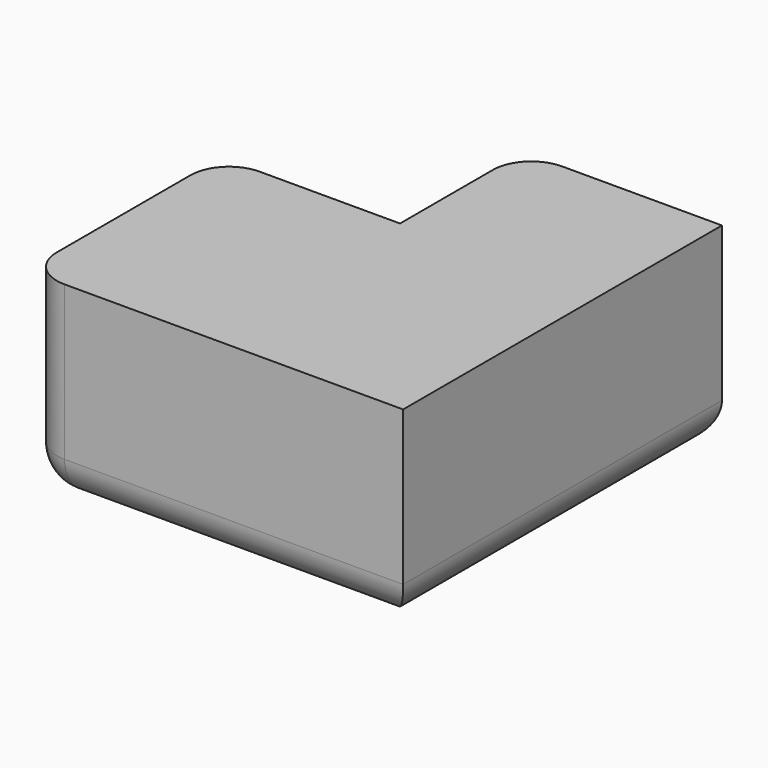
from build123d import *

# Parameters (mm, degrees)
F0_W        = 23.5866680741
F0_H        = 16.0968005657
F0_W_2      = 26.164457202
F0_H_2      = 20.3793495893
F1_DEPTH    = 25.4
F2_R        = 5.08
F3_R        = 5.08
F4_T1_DEPTH = 33.02
F4_S5_W     = 5.08
F4_S5_H     = 5.08
F4_T6_DEPTH = 5.08


# Not quite as in the source:
# - a fillet or chamfer that OpenCascade refuses, or shapes differently, is made with other operations: its cross-section is extruded or revolved along the edge and cut away or added


with BuildPart() as f1:
    # F0 (on Top) → F1 (new body)
    with BuildSketch(Plane.XY):
        with Locations((-11.7933340371, -6.5704584122)):
            Rectangle(F0_W, F0_H)
        with Locations((13.082228601, 9.5263421535)):
            Rectangle(F0_W_2, F0_H)
        with Locations((-11.7933340371, 9.5263421535)):
            Rectangle(F0_W, F0_H)
        with Locations((13.082228601, 27.7644172311)):
            Rectangle(F0_W_2, F0_H_2)
        with Locations((13.082228601, -6.5704584122)):
            Rectangle(F0_W_2, F0_H)
    extrude(amount=F1_DEPTH)

    # F2
    f2_edges = [f1.edges().sort_by_distance(p)[0] for p in [
        (-23.586668, 1.477942, 0),
    ]]
    fillet(f2_edges, radius=F2_R)

    # F3
    f3_edges = [f1.edges().sort_by_distance(p)[0] for p in [
        (3.828895, -14.618859, 0),
        (-18.506668, 1.477942, 0),
        (26.164457, 11.667617, 0),
        (-9.253334, 17.574742, 0),
        (13.082229, 37.954092, 0),
        (0, 27.764417, 0),
    ]]
    fillet(f3_edges, radius=F3_R)

    # F4: fillet of radius 5.08 on 1 edges, made by hand

    # F4_s2 → F4_t1 (cut)
    with BuildSketch(Plane.XY.offset(5.08)):
        with BuildLine():
            ThreePointArc((5.08, 37.9540920258), (1.4878975516, 36.4661944742), (0, 32.8740920258))
            Line((0, 32.8740920258), (0, 37.9540920258))
            Line((0, 37.9540920258), (5.08, 37.9540920258))
        make_face()
    extrude(amount=F4_T1_DEPTH, mode=Mode.SUBTRACT)


with BuildPart() as f4_tool4:
    # F4_s5 → F4_t6 (new body)
    with BuildSketch(Plane.XZ.offset(-32.8740920258)):
        with Locations((2.54, 2.54)):
            Rectangle(F4_S5_W, F4_S5_H)
    extrude(amount=-F4_T6_DEPTH)

    # F4_s7 → F4_t8 (revolve, cut)
    with BuildSketch(Plane(origin=(5.08, 32.8740920258, 5.08), x_dir=(0.7071067812, 0, 0.7071067812), z_dir=(-0.7071067812, 0, 0.7071067812))):
        with BuildLine():
            ThreePointArc((0, -5.08), (5.08, 0), (0, 5.08))
            Line((0, 5.08), (0, -5.08))
        make_face()
    revolve(axis=Axis((5.08, 32.8740920258, 5.08), (0, 1, 0)), mode=Mode.SUBTRACT)


with BuildPart() as f1_1:
    add(f1.part)

    # F4_t3: cut F4_tool4
    add(f4_tool4.part, mode=Mode.SUBTRACT)


solid = f1_1.part
